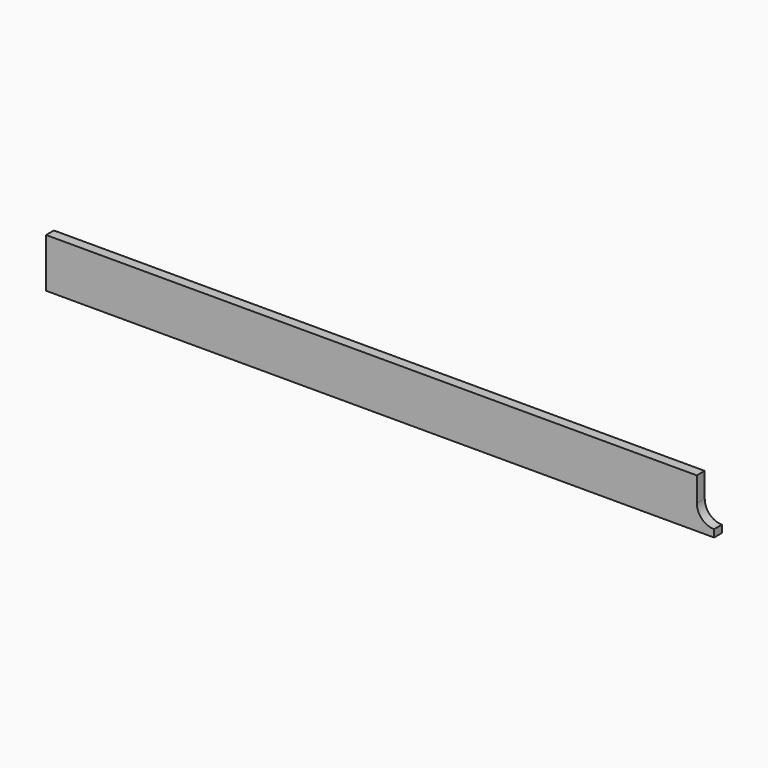
from build123d import *

# Parameters (mm, degrees)
F1_DEPTH = 50


# Not quite as in the source:
# - a feature of the source that left no trace in its solid (it failed there, or was rolled back) is left out


with BuildPart() as f1:
    # F0 (on Front) → F1 (new body)
    with BuildSketch(Plane.XZ):
        with BuildLine():
            Line((-3400, 0), (0, 0))
            Line((0, 0), (0, 37.5))
            ThreePointArc((0, 37.5), (-61.8718433538, 63.1281566462), (-87.5, 125))
            Line((-87.5, 125), (-87.5, 250))
            Line((-87.5, 250), (-3400, 250))
            Line((-3400, 250), (-3400, 0))
        make_face()
    extrude(amount=-F1_DEPTH)


solid = f1.part
